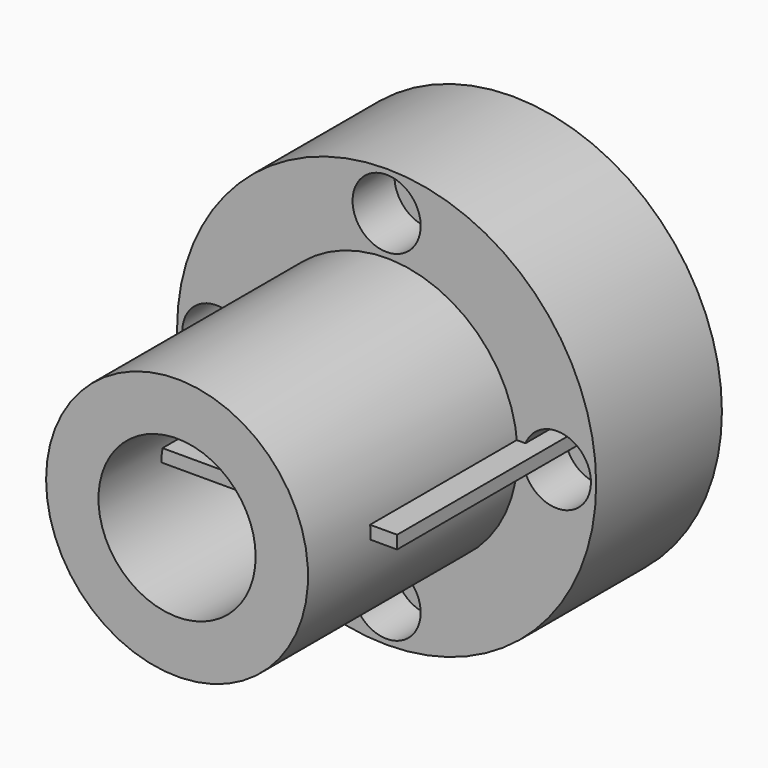
from build123d import *

# Parameters (mm, degrees)
F0_R            = 9.525
F1_DEPTH        = 31.75
F2_DEPTH        = 19.05
F3_D            = 4.9784
F3_CBORE_D      = 8.255
F3_CBORE_DEPTH  = 6.35
F3_COPIES_COUNT = 4
F4_W            = 33.3682782948
F4_H            = 27.6242401451
F4_R            = 1.524
F5_DEPTH        = 1.524
F6_W            = 38.1
F6_H            = 44.45
F6_R            = 1.6256
F7_DEPTH        = 1.5748


# Not quite as in the source:
# - a pattern or mirror of a feature is missing from the dataset's text; its kind, count and spacing are read off the source's solid


with BuildPart() as f1:
    # F0 (on Front) → F1 (new body)
    with BuildSketch(Plane.XZ):
        with BuildLine():
            ThreePointArc((15.875, 0), (0, 15.875), (-15.875, 0))
            ThreePointArc((-15.875, 0), (0, -15.875), (15.875, 0))
        make_face()
        Circle(F0_R, mode=Mode.SUBTRACT)
    extrude(amount=F1_DEPTH)

    # F0 (on Front) → F2 (join)
    with BuildSketch(Plane.XZ):
        with BuildLine():
            ThreePointArc((-25.4, 0), (0, -25.4), (25.4, 0))
            ThreePointArc((25.4, 0), (0, 25.4), (-25.4, 0))
        make_face()
        with BuildLine():
            ThreePointArc((15.875, 0), (0, -15.875), (-15.875, 0))
            ThreePointArc((-15.875, 0), (0, 15.875), (15.875, 0))
        make_face(mode=Mode.SUBTRACT)
        with BuildLine():
            ThreePointArc((15.875, 0), (0, 15.875), (-15.875, 0))
            ThreePointArc((-15.875, 0), (0, -15.875), (15.875, 0))
        make_face()
        Circle(F0_R, mode=Mode.SUBTRACT)
    extrude(amount=-F2_DEPTH)

    # F3 (through all)
    with Locations(Plane.XZ):
        with Locations((-20.6375, 0)):
            f3 = CounterBoreHole(F3_D / 2, F3_CBORE_D / 2, F3_CBORE_DEPTH)

    # F3_copies: F3 ×4 about axis
    f3_copies_axis = Axis((0, 0, 0), (0, 1, 0))
    for i in range(1, F3_COPIES_COUNT):
        add(f3.rotate(f3_copies_axis, i * 360 / F3_COPIES_COUNT), mode=Mode.SUBTRACT)


with BuildPart() as f5:
    # F4 (on Right) → F5 (new body)
    with BuildSketch(Plane.YZ):
        Rectangle(F4_W, F4_H)
        with Locations((-12.4968, 0)):
            Circle(F4_R, mode=Mode.SUBTRACT)
        with BuildLine():
            ThreePointArc((-9.6913823079, 3.648633518), (-9.3440955535, 4.9447253304), (-8.128, 5.5118))
            Line((-8.128, 5.5118), (8.128, 5.5118))
            ThreePointArc((8.128, 5.5118), (9.2505320151, 5.0468320151), (9.7155, 3.9243))
            ThreePointArc((9.7155, 3.9243), (9.7094590832, 3.7859402584), (9.6913823079, 3.648633518))
            Line((9.6913823079, 3.648633518), (8.3074623671, -4.199966482))
            ThreePointArc((8.3074623671, -4.199966482), (7.7645053896, -5.1403955535), (6.7440800592, -5.5118))
            Line((6.7440800592, -5.5118), (-6.7440800592, -5.5118))
            ThreePointArc((-6.7440800592, -5.5118), (-7.7645053896, -5.1403955535), (-8.3074623671, -4.199966482))
            Line((-8.3074623671, -4.199966482), (-9.6913823079, 3.648633518))
        make_face(mode=Mode.SUBTRACT)
        with Locations((12.4968, 0)):
            Circle(F4_R, mode=Mode.SUBTRACT)
    extrude(amount=F5_DEPTH)


with BuildPart() as f7:
    # F6 (on Top) → F7 (new body)
    with BuildSketch(Plane.XY):
        Rectangle(F6_W, F6_H)
        with Locations((0, -19.9898)):
            Circle(F6_R, mode=Mode.SUBTRACT)
        with BuildLine():
            Line((-6.50875, 14.2875), (6.50875, 14.2875))
            ThreePointArc((6.50875, 14.2875), (9.3150800378, 13.1250800378), (10.4775, 10.31875))
            Line((10.4775, 10.31875), (10.4775, -10.31875))
            ThreePointArc((10.4775, -10.31875), (9.3150800378, -13.1250800378), (6.50875, -14.2875))
            Line((6.50875, -14.2875), (-6.50875, -14.2875))
            ThreePointArc((-6.50875, -14.2875), (-9.3150800378, -13.1250800378), (-10.4775, -10.31875))
            Line((-10.4775, -10.31875), (-10.4775, 10.31875))
            ThreePointArc((-10.4775, 10.31875), (-9.3150800378, 13.1250800378), (-6.50875, 14.2875))
        make_face(mode=Mode.SUBTRACT)
        with Locations((0, 19.9898)):
            Circle(F6_R, mode=Mode.SUBTRACT)
    extrude(amount=F7_DEPTH)


solid = Compound([f1.part, f5.part, f7.part])
